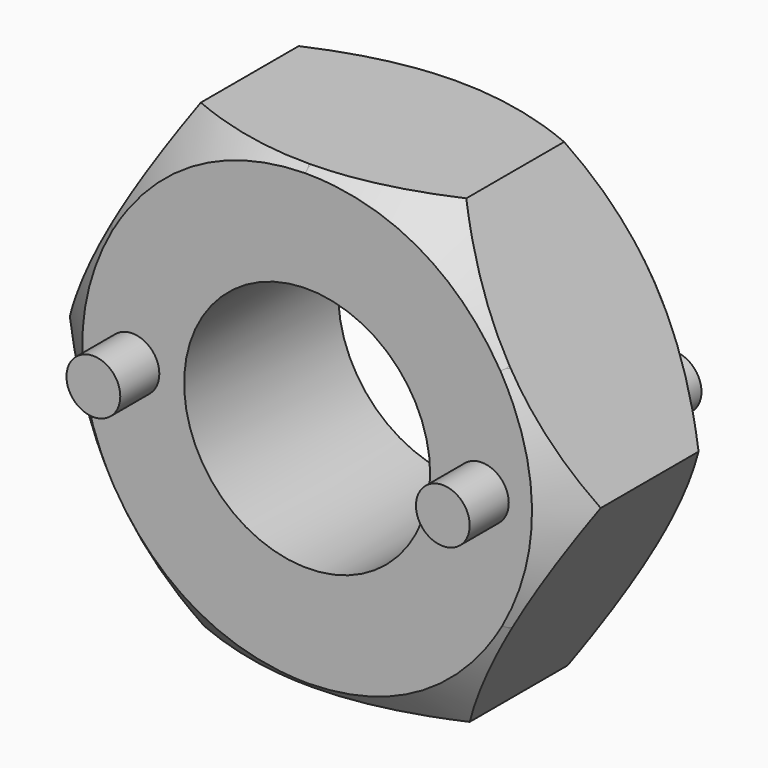
from build123d import *

# Parameters (mm, degrees)
F0_R          = 1.3716
F0_R_2        = 6.7945
F1_DEPTH      = 10.63938
F2_R          = 1.4859
F3_DEPTH      = 13.335
F3_DEPTH_BACK = 2.667
F4_SIZE2      = 0.3175
F4_SIZE       = 0.3175
F5_T1_DEPTH   = 34.0860309116
F5_T3_DEPTH   = 34.0860309116
F5_T5_DEPTH   = 34.0860309116
F5_T7_DEPTH   = 34.0860309116
F5_T9_DEPTH   = 34.0860309116
F5_T11_DEPTH  = 34.0860309116
F5_T13_DEPTH  = 34.0860309116
F5_T15_DEPTH  = 34.0860309116
F5_T17_DEPTH  = 34.0860309116
F5_T19_DEPTH  = 34.0860309116
F5_T21_DEPTH  = 34.0860309116
F5_T23_DEPTH  = 34.0860309116


# Not quite as in the source:
# - a fillet or chamfer that OpenCascade refuses, or shapes differently, is made with other operations: its cross-section is extruded or revolved along the edge and cut away or added


with BuildPart() as f1:
    # F0 (on Front) → F1 (new body)
    with BuildSketch(Plane.XZ):
        Polygon((7.427176254, -12.6447770335), (14.6642862631, 0.1097347976), (7.2371100092, 12.754511831), (-7.427176254, 12.6447770335), (-14.6642862631, -0.1097347976), (-7.2371100092, -12.754511831), align=None)
        with Locations((-9.652, 0)):
            Circle(F0_R, mode=Mode.SUBTRACT)
        Circle(F0_R_2, mode=Mode.SUBTRACT)
        with Locations((9.652, 0)):
            Circle(F0_R, mode=Mode.SUBTRACT)
    extrude(amount=F1_DEPTH)

    # F4
    f4_edges = [f1.edges().sort_by_distance(p)[0] for p in [
        (-11.045731, -10.63938, 6.267521),
        (-0.095033, -10.63938, 12.699644),
        (-10.950698, -10.63938, -6.432123),
        (0.095033, -10.63938, -12.699644),
        (11.045731, -10.63938, -6.267521),
        (10.950698, -10.63938, 6.432123),
        (-0.095033, 0, 12.699644),
        (10.950698, 0, 6.432123),
        (11.045731, 0, -6.267521),
        (0.095033, 0, -12.699644),
        (-10.950698, 0, -6.432123),
        (-11.045731, 0, 6.267521),
    ]]
    chamfer(f4_edges, length=F4_SIZE, length2=F4_SIZE2)

    # F5: fillet of radius 17.78 on 12 edges, made by hand

    # F5_s2 → F5_t1 (cut)
    with BuildSketch(Plane(origin=(21.2363539354, -18.3917369138, 0.158914451), x_dir=(-0.6546641443, -0.7559198755, 0), z_dir=(-0.7559077819, 0.6546536707, -0.0056565581))):
        with BuildLine():
            ThreePointArc((-7.0150486709, -6.2518889722), (-8.1325730637, 0.0398403383), (-6.9534591831, 6.3203187391))
            Line((-6.9534591831, 6.3203187391), (-9.3601778581, 0.0458542026))
            Line((-9.3601778581, 0.0458542026), (-7.0150486709, -6.2518889722))
        make_face()
    extrude(amount=F5_T1_DEPTH, mode=Mode.SUBTRACT)

    # F5_s4 → F5_t3 (cut)
    with BuildSketch(Plane(origin=(10.7558009193, -18.3917369138, -18.3117647664), x_dir=(-0.8632209447, -0.5048263073, 0), z_dir=(-0.382852614, 0.6546536707, 0.651807063))):
        with BuildLine():
            ThreePointArc((-9.343230333, -1.0005351171), (-5.4311798933, -6.0533145347), (0.0146355079, -9.3966381955))
            Line((0.0146355079, -9.3966381955), (-6.2510117502, -6.9670570718))
            Line((-6.2510117502, -6.9670570718), (-9.343230333, -1.0005351171))
        make_face()
    extrude(amount=F5_T3_DEPTH, mode=Mode.SUBTRACT)

    # F5_s6 → F5_t5 (cut)
    with BuildSketch(Plane(origin=(-10.4805530161, -18.3917369138, -18.4706792173), x_dir=(-0.8688328915, 0.49510545, 0), z_dir=(0.3730551679, 0.6546536707, 0.6574636211))):
        with BuildLine():
            ThreePointArc((-0.1757380658, -9.3950061047), (5.3265979335, -6.1455419894), (9.324702912, -1.1605770882))
            Line((9.324702912, -1.1605770882), (6.130643235, -7.0732061802))
            Line((6.130643235, -7.0732061802), (-0.1757380658, -9.3950061047))
        make_face()
    extrude(amount=F5_T5_DEPTH, mode=Mode.SUBTRACT)

    # F5_s8 → F5_t7 (cut)
    with BuildSketch(Plane(origin=(-21.2363539354, -18.3917369138, -0.158914451), x_dir=(-0.6546641443, 0.7559198755, 0), z_dir=(0.7559077819, 0.6546536707, 0.0056565581))):
        with BuildLine():
            ThreePointArc((6.9534591831, -6.3203187391), (8.1325730637, -0.0398403383), (7.0150486709, 6.2518889722))
            Line((7.0150486709, 6.2518889722), (9.3601778581, -0.0458542026))
            Line((9.3601778581, -0.0458542026), (6.9534591831, -6.3203187391))
        make_face()
    extrude(amount=F5_T7_DEPTH, mode=Mode.SUBTRACT)

    # F5_s10 → F5_t9 (cut)
    with BuildSketch(Plane(origin=(-10.7558009193, -18.3917369138, 18.3117647664), x_dir=(-0.8632209447, 0.5048263073, 0), z_dir=(0.382852614, 0.6546536707, -0.651807063))):
        with BuildLine():
            ThreePointArc((-0.0146355079, 9.3966381955), (5.4311798933, 6.0533145347), (9.343230333, 1.0005351171))
            Line((9.343230333, 1.0005351171), (6.2510117502, 6.9670570718))
            Line((6.2510117502, 6.9670570718), (-0.0146355079, 9.3966381955))
        make_face()
    extrude(amount=F5_T9_DEPTH, mode=Mode.SUBTRACT)

    # F5_s12 → F5_t11 (cut)
    with BuildSketch(Plane(origin=(10.4805530161, -18.3917369138, 18.4706792173), x_dir=(-0.8688328915, -0.49510545, 0), z_dir=(-0.3730551679, 0.6546536707, -0.6574636211))):
        with BuildLine():
            ThreePointArc((-9.324702912, 1.1605770882), (-5.3265979335, 6.1455419894), (0.1757380658, 9.3950061047))
            Line((0.1757380658, 9.3950061047), (-6.130643235, 7.0732061802))
            Line((-6.130643235, 7.0732061802), (-9.324702912, 1.1605770882))
        make_face()
    extrude(amount=F5_T11_DEPTH, mode=Mode.SUBTRACT)

    # F5_s14 → F5_t13 (cut)
    with BuildSketch(Plane(origin=(-15.9713737111, 13.8320026281, -0.1195159062), x_dir=(0.6546641443, 0.7559198755, 0), z_dir=(0.7559077819, -0.6546536707, 0.0056565581))):
        with BuildLine():
            ThreePointArc((-14.9959779879, -6.3597179142), (-16.1750918685, -0.0792395135), (-15.0575674756, 6.2124897971))
            Line((-15.0575674756, 6.2124897971), (-17.4026966628, -0.0852533777))
            Line((-17.4026966628, -0.0852533777), (-14.9959779879, -6.3597179142))
        make_face()
    extrude(amount=F5_T13_DEPTH, mode=Mode.SUBTRACT)

    # F5_s16 → F5_t15 (cut)
    with BuildSketch(Plane(origin=(-7.8821830446, 13.8320026281, -13.8913733202), x_dir=(0.8688328915, 0.49510545, 0), z_dir=(0.3730551679, -0.6546536707, 0.6574636211))):
        with BuildLine():
            ThreePointArc((-5.0918769572, -15.4724967867), (-10.5942129565, -12.2230326714), (-14.592317935, -7.2380677702))
            Line((-14.592317935, -7.2380677702), (-11.3982582579, -13.1506968622))
            Line((-11.3982582579, -13.1506968622), (-5.0918769572, -15.4724967867))
        make_face()
    extrude(amount=F5_T15_DEPTH, mode=Mode.SUBTRACT)

    # F5_s18 → F5_t17 (cut)
    with BuildSketch(Plane(origin=(-8.0891906664, 13.8320026281, 13.771857414), x_dir=(0.8632209447, 0.5048263073, 0), z_dir=(0.382852614, -0.6546536707, -0.651807063))):
        with BuildLine():
            ThreePointArc((-14.7142692504, 6.9868196047), (-10.8022188107, 12.0395990224), (-5.3564034095, 15.3829226832))
            Line((-5.3564034095, 15.3829226832), (-11.6220506676, 12.9533415595))
            Line((-11.6220506676, 12.9533415595), (-14.7142692504, 6.9868196047))
        make_face()
    extrude(amount=F5_T17_DEPTH, mode=Mode.SUBTRACT)

    # F5_s20 → F5_t19 (cut)
    with BuildSketch(Plane(origin=(7.8821830446, 13.8320026281, 13.8913733202), x_dir=(0.8688328915, -0.49510545, 0), z_dir=(-0.3730551679, -0.6546536707, -0.6574636211))):
        with BuildLine():
            ThreePointArc((14.592317935, 7.2380677702), (10.5942129565, 12.2230326714), (5.0918769572, 15.4724967867))
            Line((5.0918769572, 15.4724967867), (11.3982582579, 13.1506968622))
            Line((11.3982582579, 13.1506968622), (14.592317935, 7.2380677702))
        make_face()
    extrude(amount=F5_T19_DEPTH, mode=Mode.SUBTRACT)

    # F5_s22 → F5_t21 (cut)
    with BuildSketch(Plane(origin=(15.9713737111, 13.8320026281, 0.1195159062), x_dir=(0.6546641443, -0.7559198755, 0), z_dir=(-0.7559077819, -0.6546536707, -0.0056565581))):
        with BuildLine():
            ThreePointArc((15.0575674756, -6.2124897971), (16.1750918685, 0.0792395135), (14.9959779879, 6.3597179142))
            Line((14.9959779879, 6.3597179142), (17.4026966628, 0.0852533777))
            Line((17.4026966628, 0.0852533777), (15.0575674756, -6.2124897971))
        make_face()
    extrude(amount=F5_T21_DEPTH, mode=Mode.SUBTRACT)

    # F5_s24 → F5_t23 (cut)
    with BuildSketch(Plane(origin=(8.0891906664, 13.8320026281, -13.771857414), x_dir=(0.8632209447, -0.5048263073, 0), z_dir=(-0.382852614, -0.6546536707, 0.651807063))):
        with BuildLine():
            ThreePointArc((14.7142692504, -6.9868196047), (10.8022188107, -12.0395990224), (5.3564034095, -15.3829226832))
            Line((5.3564034095, -15.3829226832), (11.6220506676, -12.9533415595))
            Line((11.6220506676, -12.9533415595), (14.7142692504, -6.9868196047))
        make_face()
    extrude(amount=F5_T23_DEPTH, mode=Mode.SUBTRACT)


with BuildPart() as f3:
    # F2 (on Front) → F3 (new body, two sides)
    with BuildSketch(Plane.XZ) as f3_sk:
        with Locations((9.652, 0)):
            Circle(F2_R)
    extrude(amount=F3_DEPTH)
    extrude(f3_sk.sketch, amount=-F3_DEPTH_BACK)


with BuildPart() as f3b:
    # F2 (on Front) → F3, piece 2 (new body, two sides)
    with BuildSketch(Plane.XZ) as f3_2_sk:
        with Locations((-9.652, 0)):
            Circle(F2_R)
    extrude(amount=F3_DEPTH)
    extrude(f3_2_sk.sketch, amount=-F3_DEPTH_BACK)


solid = Compound([f1.part, f3.part, f3b.part])
